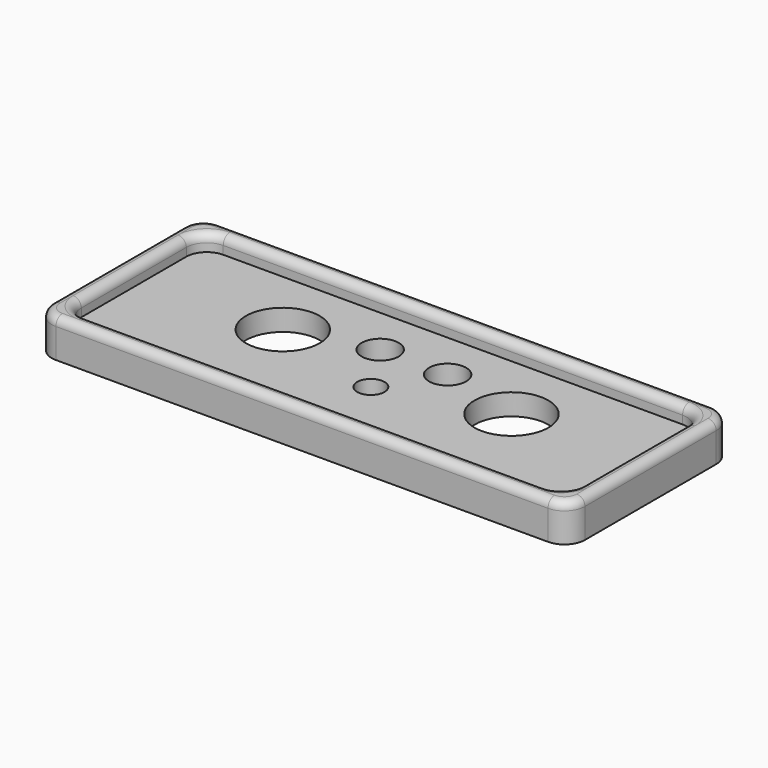
from build123d import *

# Parameters (mm, degrees)
F1_DEPTH = 3.302
F2_DEPTH = 2.54
F3_R     = 5.715
F3_R_2   = 2.8702
F3_R_3   = 2.1123361497
F4_DEPTH = 3.303
F5_R     = 1.26999


# Not quite as in the source:
# - a fillet or chamfer is up to 0.001 mm smaller than in the source, because OpenCascade refuses the exact size


with BuildPart() as f1:
    # F0 (on Top) → F1 (new body)
    with BuildSketch(Plane.XY):
        with BuildLine():
            Line((86.5189202702, -3.8629329861), (10.3189202702, -3.8629329861))
            ThreePointArc((10.3189202702, -3.8629329861), (8.0738562399, -4.7928689558), (7.1439202702, -7.0379329861))
            Line((7.1439202702, -7.0379329861), (7.1439202702, -32.4379329861))
            ThreePointArc((7.1439202702, -32.4379329861), (8.0738562399, -34.6829970164), (10.3189202702, -35.6129329861))
            Line((10.3189202702, -35.6129329861), (86.5189202702, -35.6129329861))
            ThreePointArc((86.5189202702, -35.6129329861), (88.7639843005, -34.6829970164), (89.6939202702, -32.4379329861))
            Line((89.6939202702, -32.4379329861), (89.6939202702, -7.0379329861))
            ThreePointArc((89.6939202702, -7.0379329861), (88.7639843005, -4.7928689558), (86.5189202702, -3.8629329861))
        make_face()
        with BuildLine():
            Line((83.9789202702, -33.0729329861), (12.8589202702, -33.0729329861))
            ThreePointArc((12.8589202702, -33.0729329861), (10.6138562399, -32.1429970164), (9.6839202702, -29.8979329861))
            Line((9.6839202702, -29.8979329861), (9.6839202702, -9.5779329861))
            ThreePointArc((9.6839202702, -9.5779329861), (10.6138562399, -7.3328689558), (12.8589202702, -6.4029329861))
            Line((12.8589202702, -6.4029329861), (83.9789202702, -6.4029329861))
            ThreePointArc((83.9789202702, -6.4029329861), (86.2239843005, -7.3328689558), (87.1539202702, -9.5779329861))
            Line((87.1539202702, -9.5779329861), (87.1539202702, -29.8979329861))
            ThreePointArc((87.1539202702, -29.8979329861), (86.2239843005, -32.1429970164), (83.9789202702, -33.0729329861))
        make_face(mode=Mode.SUBTRACT)
        with BuildLine():
            ThreePointArc((9.6839202702, -29.8979329861), (10.6138562399, -32.1429970164), (12.8589202702, -33.0729329861))
            Line((12.8589202702, -33.0729329861), (83.9789202702, -33.0729329861))
            ThreePointArc((83.9789202702, -33.0729329861), (86.2239843005, -32.1429970164), (87.1539202702, -29.8979329861))
            Line((87.1539202702, -29.8979329861), (87.1539202702, -9.5779329861))
            ThreePointArc((87.1539202702, -9.5779329861), (86.2239843005, -7.3328689558), (83.9789202702, -6.4029329861))
            Line((83.9789202702, -6.4029329861), (12.8589202702, -6.4029329861))
            ThreePointArc((12.8589202702, -6.4029329861), (10.6138562399, -7.3328689558), (9.6839202702, -9.5779329861))
            Line((9.6839202702, -9.5779329861), (9.6839202702, -29.8979329861))
        make_face()
    extrude(amount=-F1_DEPTH)

    # F0 (on Top) → F2 (join)
    with BuildSketch(Plane.XY):
        with BuildLine():
            Line((86.5189202702, -3.8629329861), (10.3189202702, -3.8629329861))
            ThreePointArc((10.3189202702, -3.8629329861), (8.0738562399, -4.7928689558), (7.1439202702, -7.0379329861))
            Line((7.1439202702, -7.0379329861), (7.1439202702, -32.4379329861))
            ThreePointArc((7.1439202702, -32.4379329861), (8.0738562399, -34.6829970164), (10.3189202702, -35.6129329861))
            Line((10.3189202702, -35.6129329861), (86.5189202702, -35.6129329861))
            ThreePointArc((86.5189202702, -35.6129329861), (88.7639843005, -34.6829970164), (89.6939202702, -32.4379329861))
            Line((89.6939202702, -32.4379329861), (89.6939202702, -7.0379329861))
            ThreePointArc((89.6939202702, -7.0379329861), (88.7639843005, -4.7928689558), (86.5189202702, -3.8629329861))
        make_face()
        with BuildLine():
            Line((83.9789202702, -33.0729329861), (12.8589202702, -33.0729329861))
            ThreePointArc((12.8589202702, -33.0729329861), (10.6138562399, -32.1429970164), (9.6839202702, -29.8979329861))
            Line((9.6839202702, -29.8979329861), (9.6839202702, -9.5779329861))
            ThreePointArc((9.6839202702, -9.5779329861), (10.6138562399, -7.3328689558), (12.8589202702, -6.4029329861))
            Line((12.8589202702, -6.4029329861), (83.9789202702, -6.4029329861))
            ThreePointArc((83.9789202702, -6.4029329861), (86.2239843005, -7.3328689558), (87.1539202702, -9.5779329861))
            Line((87.1539202702, -9.5779329861), (87.1539202702, -29.8979329861))
            ThreePointArc((87.1539202702, -29.8979329861), (86.2239843005, -32.1429970164), (83.9789202702, -33.0729329861))
        make_face(mode=Mode.SUBTRACT)
    extrude(amount=F2_DEPTH)

    # F3 (on Top) → F4 (cut, through all)
    with BuildSketch(Plane.XY):
        with Locations((30.7151202702, -17.1979329861)):
            Circle(F3_R)
        with BuildLine():
            ThreePointArc((71.8377202702, -17.1979329861), (66.1227202702, -11.4829329861), (60.4077202702, -17.1979329861))
            ThreePointArc((60.4077202702, -17.1979329861), (66.1227202702, -22.9129329861), (71.8377202702, -17.1979329861))
        make_face()
        with Locations((43.1992202702, -13.949079439)):
            Circle(F3_R_2)
        with BuildLine():
            ThreePointArc((56.5088202702, -13.949079439), (53.6386202702, -11.078879439), (50.7684202702, -13.949079439))
            ThreePointArc((50.7684202702, -13.949079439), (53.6386202702, -16.819279439), (56.5088202702, -13.949079439))
        make_face()
        with Locations((48.4189202702, -22.2779329861)):
            Circle(F3_R_3)
    extrude(amount=-F4_DEPTH, mode=Mode.SUBTRACT)

    # F5 (radius 1.27 in the source; OpenCascade refuses exactly that, so slightly less here)
    f5_edges = [f1.edges().sort_by_distance(p)[0] for p in [
        (48.41892, -6.402933, 2.54),
        (10.613856, -7.332869, 2.54),
        (9.68392, -19.737933, 2.54),
        (10.613856, -32.142997, 2.54),
        (48.41892, -33.072933, 2.54),
        (87.15392, -19.737933, 2.54),
        (86.223984, -7.332869, 2.54),
        (86.223984, -32.142997, 2.54),
        (7.14392, -19.737933, 2.54),
        (8.073856, -4.792869, 2.54),
    ]]
    fillet(f5_edges, radius=F5_R)


solid = f1.part
